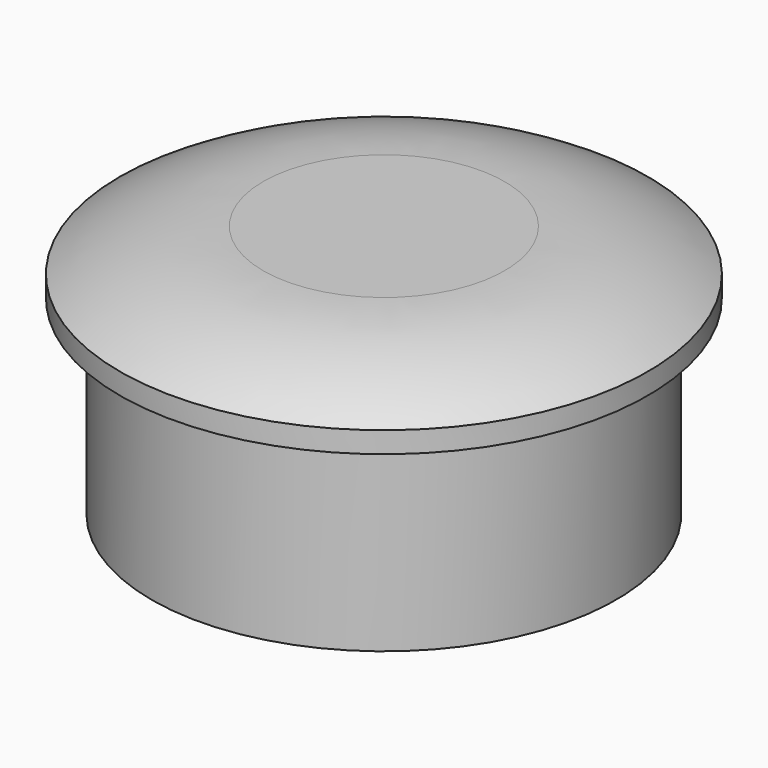
from build123d import *

# Parameters (mm, degrees)
F3_DEPTH = 1


# Not quite as in the source:
# - a fillet or chamfer that OpenCascade refuses, or shapes differently, is made with other operations: its cross-section is extruded or revolved along the edge and cut away or added


with BuildPart() as f1:
    # F0 (on Front) → F1 (revolve)
    with BuildSketch(Plane.XZ):
        Polygon((0, 7.2039468596), (0, 10.2039468596), (-12.5, 10.2039468596), (-12.5, 8.2039468596), (-11, 8.2039468596), (-11, -1.7960531404), (-9, -1.853223308), (-9, 7.2039468596), align=None)
    revolve(axis=Axis((0, 0, 8.7039468596), (0, 0, -1)))

    # F2: fillet of radius 12.5 on 1 edges, made by hand

    # F2_s1 → F2_t2 (revolve, cut)
    with BuildSketch(Plane.XZ):
        with BuildLine():
            ThreePointArc((-5.7176700169, 10.2039468596), (-9.2532039228, 9.6935256679), (-12.5, 8.2039468596))
            Line((-12.5, 8.2039468596), (-12.6356465997, 8.4139468596))
            ThreePointArc((-12.6356465997, 8.4139468596), (-12.75, 9.2039468596), (-12.75, 10.2039468596))
            Line((-12.75, 10.2039468596), (-12.5, 10.4539468596))
            Line((-12.5, 10.4539468596), (-5.7176700169, 10.4539468596))
            Line((-5.7176700169, 10.4539468596), (-5.7176700169, 10.2039468596))
        make_face()
    revolve(axis=Axis((0, 0, 10.2039468596), (0, 0, -1)), mode=Mode.SUBTRACT)

    # F3 (add): a face of the model
    f3_faces = [f1.faces().sort_by_distance(p)[0] for p in [
        (12.1464466094, 0, 8.2039468596),
    ]]
    extrude(f3_faces, amount=F3_DEPTH)


solid = f1.part
